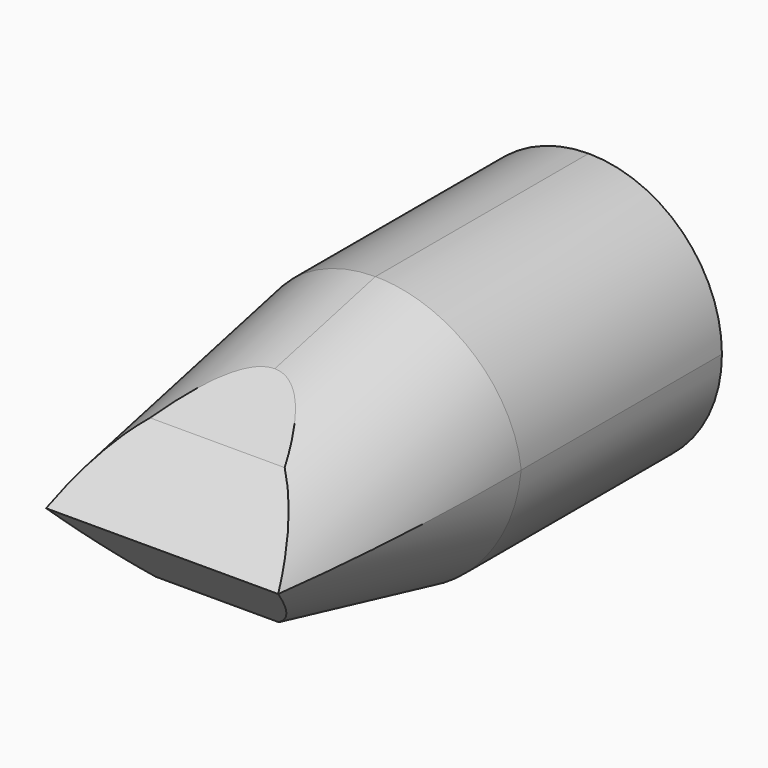
from build123d import *

# Parameters (mm, degrees)
F0_W        = 50.8
F0_H        = 25.4
F1_DEPTH    = 25.4
F3_DEPTH    = 25.4
F4_T1_DEPTH = 161.5415732481
F4_T3_DEPTH = 111.125
F4_T5_DEPTH = 161.5415732481


# Not quite as in the source:
# - a fillet or chamfer that OpenCascade refuses, or shapes differently, is made with other operations: its cross-section is extruded or revolved along the edge and cut away or added


with BuildPart() as f1:
    # F0 (on Right) → F1 (new body)
    with BuildSketch(Plane.YZ):
        Rectangle(F0_W, F0_H)
    extrude(amount=F1_DEPTH)

    # F2 (on face) → F3 (cut)
    with BuildSketch(Plane.YZ.offset(25.4)):
        Polygon((-11.9801070541, 9.8408022895), (0, 12.7), (-25.4, 12.7), (-25.4, 0), (-18.8258830458, 6.4179147594), align=None)
        Polygon((-18.8258830458, -6.7341208707), (-25.4, 0), (-25.4, -12.7), (0, -12.7), (-11.9801070541, -9.8408022895), align=None)
    extrude(amount=-F3_DEPTH, mode=Mode.SUBTRACT)

    # F4: fillet of radius 12.7 on 16 edges, made by hand

    # F4_s2 → F4_t1 (cut)
    with BuildSketch(Plane(origin=(0, -101.7603840671, -24.28634868), x_dir=(1, 0, 0), z_dir=(0, 0.9726818339, 0.2321423056))):
        with BuildLine():
            ThreePointArc((25.4, 0.3469407097), (21.6802561211, -8.6333154114), (12.7, -12.3530592903))
            Line((12.7, -12.3530592903), (25.4, -12.3530592903))
            Line((25.4, -12.3530592903), (25.4, 0.3469407097))
        make_face()
        with BuildLine():
            ThreePointArc((0, 0.3469407097), (3.7197438789, -8.6333154114), (12.7, -12.3530592903))
            Line((12.7, -12.3530592903), (0, -12.3530592903))
            Line((0, -12.3530592903), (0, 0.3469407097))
        make_face()
    extrude(amount=F4_T1_DEPTH, mode=Mode.SUBTRACT)

    # F4_s4 → F4_t3 (cut)
    with BuildSketch(Plane.XZ.offset(-57.15)):
        with BuildLine():
            ThreePointArc((12.7, 12.7), (21.6802561211, 8.9802561211), (25.4, 0))
            Line((25.4, 0), (25.4, 12.7))
            Line((25.4, 12.7), (12.7, 12.7))
        make_face()
        with BuildLine():
            ThreePointArc((12.7, -12.7), (21.6802561211, -8.9802561211), (25.4, 0))
            Line((25.4, 0), (25.4, -12.7))
            Line((25.4, -12.7), (12.7, -12.7))
        make_face()
        with BuildLine():
            ThreePointArc((12.7, -12.7), (3.7197438789, -8.9802561211), (0, 0))
            Line((0, 0), (0, -12.7))
            Line((0, -12.7), (12.7, -12.7))
        make_face()
        with BuildLine():
            ThreePointArc((12.7, 12.7), (3.7197438789, 8.9802561211), (0, 0))
            Line((0, 0), (0, 12.7))
            Line((0, 12.7), (12.7, 12.7))
        make_face()
    extrude(amount=F4_T3_DEPTH, mode=Mode.SUBTRACT)

    # F4_s6 → F4_t5 (cut)
    with BuildSketch(Plane(origin=(0, 55.3681696483, -13.2142845782), x_dir=(1, 0, 0), z_dir=(0, -0.9726818339, 0.2321423056))):
        with BuildLine():
            ThreePointArc((25.4, 0.3469407097), (21.6802561211, -8.6333154114), (12.7, -12.3530592903))
            Line((12.7, -12.3530592903), (25.4, -12.3530592903))
            Line((25.4, -12.3530592903), (25.4, 0.3469407097))
        make_face()
        with BuildLine():
            ThreePointArc((0, 0.3469407097), (3.7197438789, -8.6333154114), (12.7, -12.3530592903))
            Line((12.7, -12.3530592903), (0, -12.3530592903))
            Line((0, -12.3530592903), (0, 0.3469407097))
        make_face()
    extrude(amount=F4_T5_DEPTH, mode=Mode.SUBTRACT)


solid = f1.part
